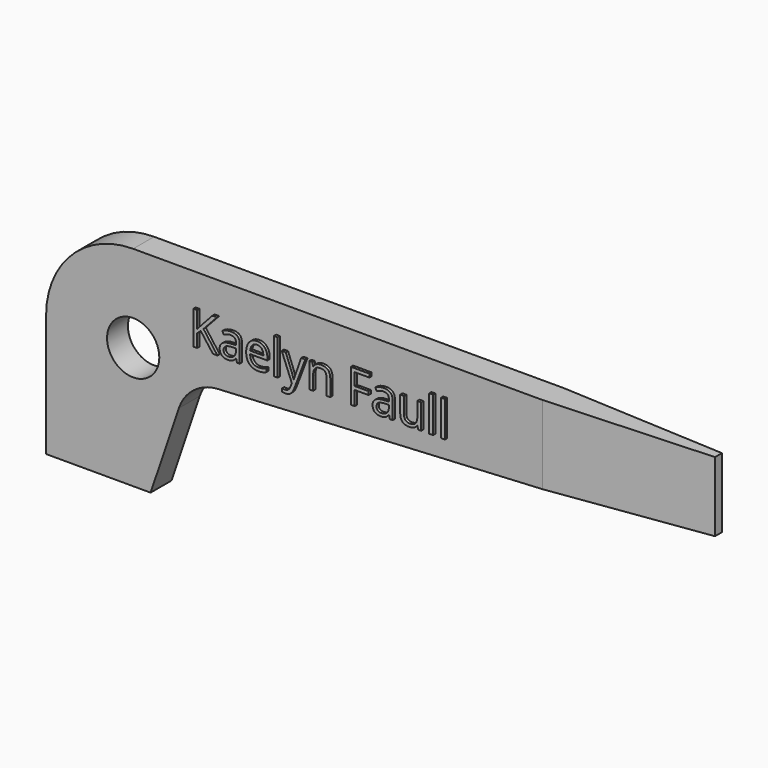
from build123d import *

# Parameters (mm, degrees)
F1_DEPTH     = 2.38125
F2_R         = 2.38125
F3_DEPTH     = 2.38225
F5_DEPTH     = 25.4
F6_TEXT_SIZE = 4.2704891206
F7_DEPTH     = 0.254


# Not quite as in the source:
# - Text() gives the source's letters only with a copy of the font that has no kerning and outlines rounded to 1/6400 em; it was checked with that copy


with BuildPart() as f1:
    # F0 (on Front) → F1 (new body)
    with BuildSketch(Plane.XZ):
        with BuildLine():
            Line((60.325, 19.05), (7.9375, 19.05))
            ThreePointArc((7.9375, 19.05), (2.3248399243, 16.7251600757), (0, 11.1125))
            Line((0, 11.1125), (0, 0))
            Line((0, 0), (9.525, 0))
            Line((9.525, 0), (12.100344796, 7.6142740092))
            ThreePointArc((12.100344796, 7.6142740092), (13.4681285679, 9.5097542378), (15.6631963617, 10.3130942181))
            Line((15.6631963617, 10.3130942181), (60.325, 12.7))
            Line((60.325, 12.7), (60.325, 19.05))
        make_face()
    extrude(amount=F1_DEPTH)

    # F2 (on face) → F3 (cut, through all)
    with BuildSketch(Plane.XZ.offset(2.38125)):
        with Locations((7.9375, 11.1125)):
            Circle(F2_R)
    extrude(amount=-F3_DEPTH, mode=Mode.SUBTRACT)

    # F4 (on face) → F5 (cut)
    with BuildSketch(Plane.XY.offset(19.05)):
        Polygon((60.325, -2.38125), (60.325, -1.5875), (45.24375, -2.38125), align=None)
        Polygon((60.325, 0), (45.24375, 0), (60.325, -0.79375), align=None)
    extrude(amount=-F5_DEPTH, mode=Mode.SUBTRACT)

    # F6 (on face) → F7 (join)
    with BuildSketch(Plane.XZ.offset(2.38125)):
        with Locations((13.2030602545, 13.1536871195)):
            Text('Kaelyn Faull', F6_TEXT_SIZE, font='Open Sans', text_align=(TextAlign.LEFT, TextAlign.BOTTOM))
    extrude(amount=F7_DEPTH)


solid = f1.part
